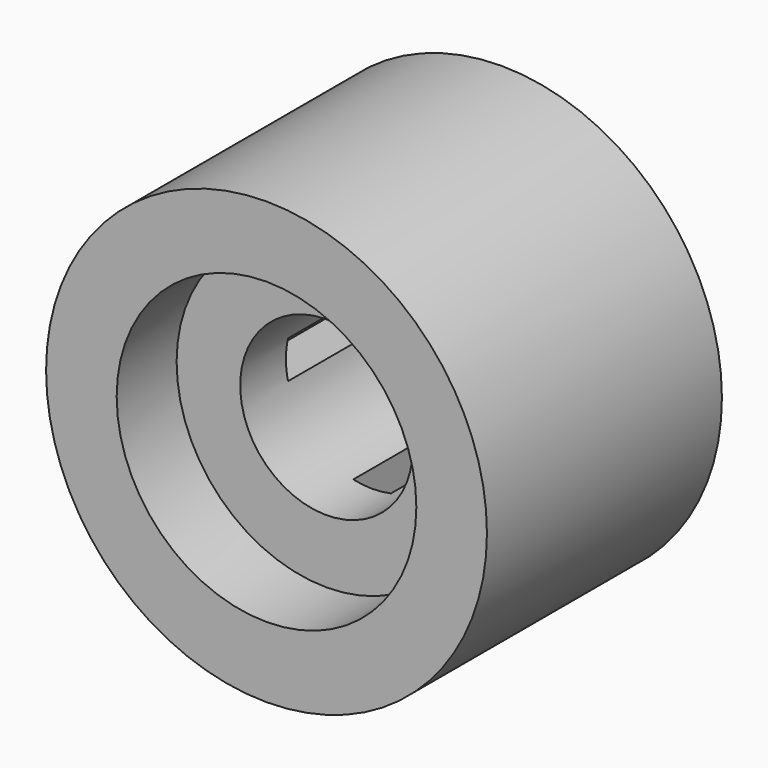
from build123d import *

# Parameters (mm, degrees)
F0_R     = 4.09
F0_R_2   = 1.6
F1_DEPTH = 5.45
F2_R     = 2.78
F3_DEPTH = 1.39
F5_DEPTH = 3


with BuildPart() as f1:
    # F0 (on Front) → F1 (new body)
    with BuildSketch(Plane.XZ):
        Circle(F0_R)
        Circle(F0_R_2, mode=Mode.SUBTRACT)
    extrude(amount=F1_DEPTH)

    # F2 (on face) → F3 (cut)
    with BuildSketch(Plane.XZ.offset(5.45)):
        Circle(F2_R)
    extrude(amount=-F3_DEPTH, mode=Mode.SUBTRACT)

    # F4 (on face) → F5 (cut)
    with BuildSketch(Plane(origin=(0, 0, 0), x_dir=(-1, 0, 0), z_dir=(0, 1, 0))):
        with BuildLine():
            Line((-0.35, 2.3612494996), (-0.35, 1.5612494996))
            ThreePointArc((-0.35, 1.5612494996), (0, 1.6), (0.35, 1.5612494996))
            Line((0.35, 1.5612494996), (0.35, 2.3612494996))
            Line((0.35, 2.3612494996), (-0.35, 2.3612494996))
        make_face()
        with BuildLine():
            Line((2.3612494996, 0.35), (1.5612494996, 0.35))
            ThreePointArc((1.5612494996, 0.35), (1.5902828678, 0.1760693054), (1.6, 0))
            ThreePointArc((1.6, 0), (1.5902828678, -0.1760693054), (1.5612494996, -0.35))
            Line((1.5612494996, -0.35), (2.3612494996, -0.35))
            Line((2.3612494996, -0.35), (2.3612494996, 0.35))
        make_face()
        with BuildLine():
            ThreePointArc((0.35, -1.5612494996), (0, -1.6), (-0.35, -1.5612494996))
            Line((-0.35, -1.5612494996), (-0.35, -2.3612494996))
            Line((-0.35, -2.3612494996), (0.35, -2.3612494996))
            Line((0.35, -2.3612494996), (0.35, -1.5612494996))
        make_face()
        with BuildLine():
            ThreePointArc((-1.5612494996, -0.35), (-1.6, 0), (-1.5612494996, 0.35))
            Line((-1.5612494996, 0.35), (-2.3612494996, 0.35))
            Line((-2.3612494996, 0.35), (-2.3612494996, -0.35))
            Line((-2.3612494996, -0.35), (-1.5612494996, -0.35))
        make_face()
    extrude(amount=-F5_DEPTH, mode=Mode.SUBTRACT)


solid = f1.part
